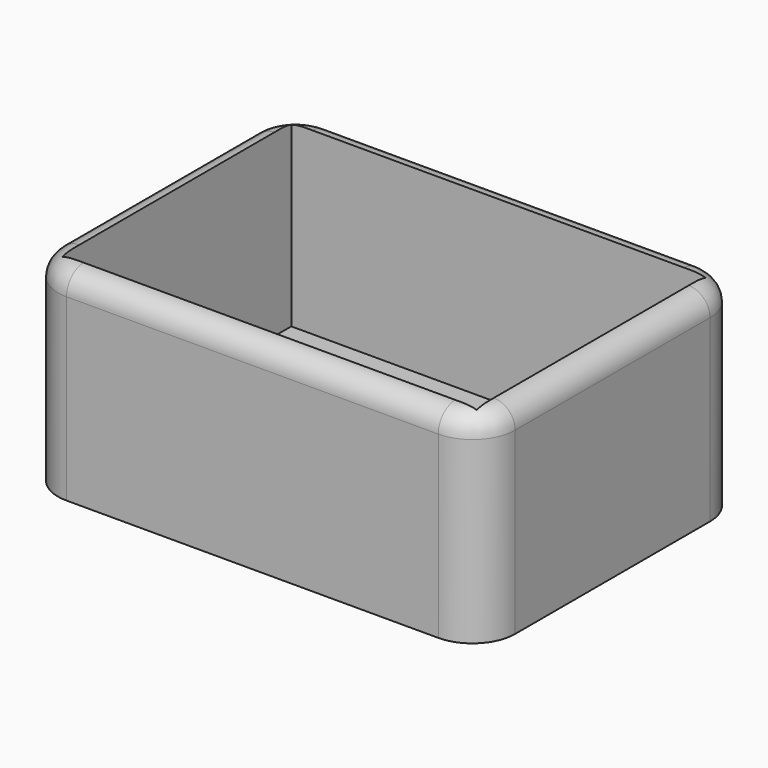
from build123d import *

# Parameters (mm, degrees)
F0_W         = 97
F0_H         = 67
F1_DEPTH     = 5
F0_W_2       = 107
F0_H_2       = 77
F2_DEPTH     = 47
F3_R         = 10
F4_T1_DEPTH  = 87
F4_T3_DEPTH  = 57
F4_T6_ANGLE  = 90
F4_T8_ANGLE  = 90
F4_T10_ANGLE = 90
F4_T12_ANGLE = 90


# Not quite as in the source:
# - a fillet or chamfer that OpenCascade refuses, or shapes differently, is made with other operations: its cross-section is extruded or revolved along the edge and cut away or added


with BuildPart() as f1:
    # F0 (on Top) → F1 (new body)
    with BuildSketch(Plane.XY):
        Rectangle(F0_W, F0_H)
    extrude(amount=F1_DEPTH)

    # F0 (on Top) → F2 (join)
    with BuildSketch(Plane.XY):
        Rectangle(F0_W_2, F0_H_2)
        Rectangle(F0_W, F0_H, mode=Mode.SUBTRACT)
    extrude(amount=F2_DEPTH)

    # F3
    f3_edges = [f1.edges().sort_by_distance(p)[0] for p in [
        (-53.5, 38.5, 23.5),
        (53.5, 38.5, 23.5),
        (53.5, -38.5, 23.5),
        (-53.5, -38.5, 23.5),
    ]]
    fillet(f3_edges, radius=F3_R)

    # F4: fillet of radius 5 on 8 edges, made by hand

    # F4_s2 → F4_t1 (cut)
    with BuildSketch(Plane.YZ.offset(-43.5)):
        with BuildLine():
            ThreePointArc((-38.5, 42), (-37.0355339059, 45.5355339059), (-33.5, 47))
            Line((-33.5, 47), (-38.5, 47))
            Line((-38.5, 47), (-38.5, 42))
        make_face()
        with BuildLine():
            ThreePointArc((38.5, 42), (37.0355339059, 45.5355339059), (33.5, 47))
            Line((33.5, 47), (38.5, 47))
            Line((38.5, 47), (38.5, 42))
        make_face()
    extrude(amount=F4_T1_DEPTH, mode=Mode.SUBTRACT)

    # F4_s4 → F4_t3 (cut)
    with BuildSketch(Plane.XZ.offset(-28.5)):
        with BuildLine():
            ThreePointArc((53.5, 42), (52.0355339059, 45.5355339059), (48.5, 47))
            Line((48.5, 47), (53.5, 47))
            Line((53.5, 47), (53.5, 42))
        make_face()
        with BuildLine():
            ThreePointArc((-53.5, 42), (-52.0355339059, 45.5355339059), (-48.5, 47))
            Line((-48.5, 47), (-53.5, 47))
            Line((-53.5, 47), (-53.5, 42))
        make_face()
    extrude(amount=F4_T3_DEPTH, mode=Mode.SUBTRACT)

    # F4_s5 → F4_t6 (revolve, cut)
    with BuildSketch(Plane.YZ.offset(43.5)):
        with BuildLine():
            ThreePointArc((38.5, 42), (37.0355339059, 45.5355339059), (33.5, 47))
            Line((33.5, 47), (38.5, 47))
            Line((38.5, 47), (38.5, 42))
        make_face()
    revolve(axis=Axis((43.5, 28.5, 47), (0, 0, -1)), revolution_arc=F4_T6_ANGLE, mode=Mode.SUBTRACT)

    # F4_s7 → F4_t8 (revolve, cut)
    with BuildSketch(Plane.YZ.offset(-43.5)):
        with BuildLine():
            ThreePointArc((38.5, 42), (37.0355339059, 45.5355339059), (33.5, 47))
            Line((33.5, 47), (38.5, 47))
            Line((38.5, 47), (38.5, 42))
        make_face()
    revolve(axis=Axis((-43.5, 28.5, 47), (0, 0, 1)), revolution_arc=F4_T8_ANGLE, mode=Mode.SUBTRACT)

    # F4_s9 → F4_t10 (revolve, cut)
    with BuildSketch(Plane.YZ.offset(43.5)):
        with BuildLine():
            ThreePointArc((-38.5, 42), (-37.0355339059, 45.5355339059), (-33.5, 47))
            Line((-33.5, 47), (-38.5, 47))
            Line((-38.5, 47), (-38.5, 42))
        make_face()
    revolve(axis=Axis((43.5, -28.5, 47), (0, 0, 1)), revolution_arc=F4_T10_ANGLE, mode=Mode.SUBTRACT)

    # F4_s11 → F4_t12 (revolve, cut)
    with BuildSketch(Plane.XZ.offset(28.5)):
        with BuildLine():
            ThreePointArc((-53.5, 42), (-52.0355339059, 45.5355339059), (-48.5, 47))
            Line((-48.5, 47), (-53.5, 47))
            Line((-53.5, 47), (-53.5, 42))
        make_face()
    revolve(axis=Axis((-43.5, -28.5, 47), (0, 0, 1)), revolution_arc=F4_T12_ANGLE, mode=Mode.SUBTRACT)


solid = f1.part
